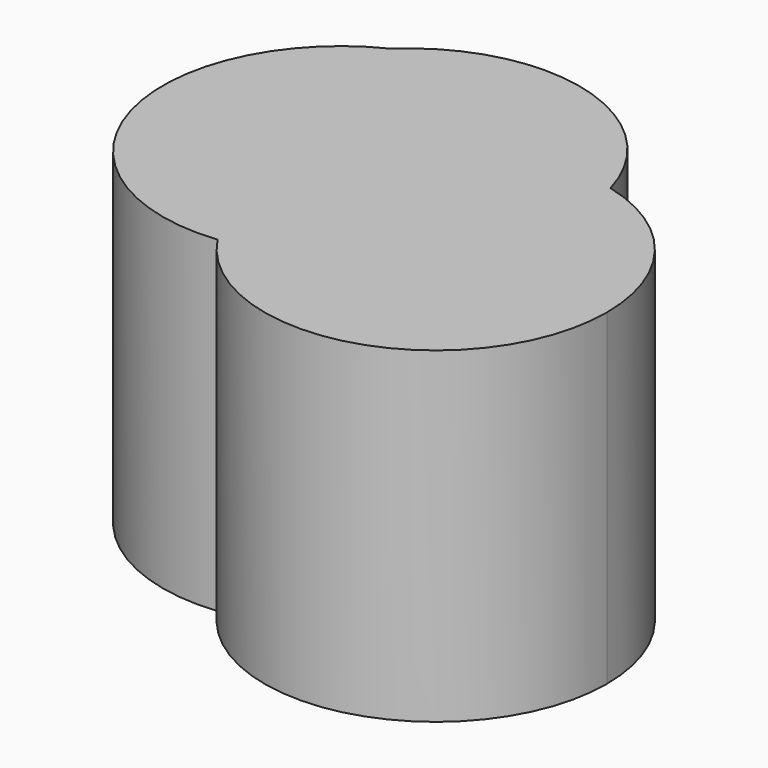
from build123d import *

# Parameters (mm, degrees)
F1_DEPTH = 71.86255


# Not quite as in the source:
# - a feature names something its author has since deleted; it is built from what else it names


with BuildPart() as f1:
    # F0 (on Top) → F1 (new body)
    with BuildSketch(Plane.XY):
        with BuildLine():
            ThreePointArc((-42.2918507094, 30.2835155285), (-36.8686969087, 30.111745716), (-31.5267122489, 29.1613237519))
            ThreePointArc((-31.5267122489, 29.1613237519), (-57.6197689064, 55.0120374135), (-93.2606175848, 46.1330223766))
            ThreePointArc((-93.2606175848, 46.1330223766), (-64.6475038211, 48.2696246863), (-42.2918507094, 30.2835155285))
        make_face()
        with BuildLine():
            ThreePointArc((-77.0032953654, -17.3475301034), (-103.8339232373, 9.6031863752), (-93.2606175848, 46.1330223766))
            ThreePointArc((-93.2606175848, 46.1330223766), (-113.8279554448, 0.2861142751), (-72.2256688216, -27.895513017))
            ThreePointArc((-72.2256688216, -27.895513017), (-75.022912939, -22.8065171242), (-77.0032953654, -17.3475301034))
        make_face()
        with BuildLine():
            ThreePointArc((-31.5267122489, 29.1613237519), (-30.4528093217, 24.0784093765), (-30.0925314228, 18.8957955688))
            ThreePointArc((-30.0925314228, 18.8957955688), (-33.4160404477, 3.4709337592), (-42.7967740776, -9.2166156752))
            ThreePointArc((-42.7967740776, -9.2166156752), (-55.3125885207, -22.0200448939), (-72.2256688216, -27.895513017))
            ThreePointArc((-72.2256688216, -27.895513017), (-30.016611499, -43.3265790466), (-3.1623770139, -7.2908688538))
            ThreePointArc((-3.1623770139, -7.2908688538), (-11.0888310752, 15.802949903), (-31.5267122489, 29.1613237519))
        make_face()
        with BuildLine():
            ThreePointArc((-42.2918507094, 30.2835155285), (-64.6475038211, 48.2696246863), (-93.2606175848, 46.1330223766))
            ThreePointArc((-93.2606175848, 46.1330223766), (-103.8339232373, 9.6031863752), (-77.0032953654, -17.3475301034))
            ThreePointArc((-77.0032953654, -17.3475301034), (-71.1589466664, 14.8569836183), (-42.2918507094, 30.2835155285))
        make_face()
        with BuildLine():
            ThreePointArc((-72.2256688216, -27.895513017), (-55.3125885207, -22.0200448939), (-42.7967740776, -9.2166156752))
            ThreePointArc((-42.7967740776, -9.2166156752), (-58.8867170827, -17.5450708199), (-77.0032953654, -17.3475301034))
            ThreePointArc((-77.0032953654, -17.3475301034), (-75.022912939, -22.8065171242), (-72.2256688216, -27.895513017))
        make_face()
        with BuildLine():
            ThreePointArc((-42.7967740776, -9.2166156752), (-33.4160404477, 3.4709337592), (-30.0925314228, 18.8957955688))
            ThreePointArc((-30.0925314228, 18.8957955688), (-30.4528093217, 24.0784093765), (-31.5267122489, 29.1613237519))
            ThreePointArc((-31.5267122489, 29.1613237519), (-36.8686969087, 30.111745716), (-42.2918507094, 30.2835155285))
            ThreePointArc((-42.2918507094, 30.2835155285), (-38.480122311, 20.9562316448), (-37.1807342965, 10.9642804431))
            ThreePointArc((-37.1807342965, 10.9642804431), (-38.6109225506, 0.4904025681), (-42.7967740776, -9.2166156752))
        make_face()
        with BuildLine():
            ThreePointArc((-77.0032953654, -17.3475301034), (-58.8867170827, -17.5450708199), (-42.7967740776, -9.2166156752))
            ThreePointArc((-42.7967740776, -9.2166156752), (-38.6109225506, 0.4904025681), (-37.1807342965, 10.9642804431))
            ThreePointArc((-37.1807342965, 10.9642804431), (-38.480122311, 20.9562316448), (-42.2918507094, 30.2835155285))
            ThreePointArc((-42.2918507094, 30.2835155285), (-71.1589466664, 14.8569836183), (-77.0032953654, -17.3475301034))
        make_face()
    extrude(amount=F1_DEPTH)


solid = f1.part
